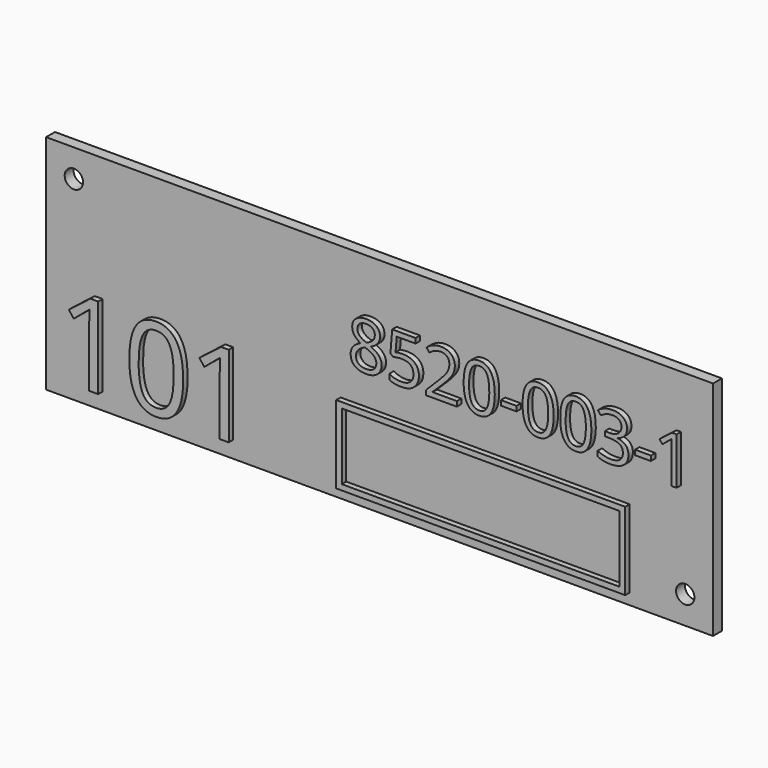
from build123d import *

# Parameters (mm, degrees)
F0_W         = 120
F0_H         = 40
F1_DEPTH     = 2
F3_D         = 3.3
F4_TEXT_SIZE = 11.8591723286
F5_DEPTH     = 1
F6_TEXT_SIZE = 20.5478077656
F7_DEPTH     = 1
F8_W         = 52
F8_H         = 14
F8_W_2       = 49.99999962
F8_H_2       = 11.99999962
F9_DEPTH     = 1


# Not quite as in the source:
# - Text() gives the source's letters only with a copy of the font that has no kerning and outlines rounded to 1/6400 em; it was checked with that copy


with BuildPart() as f1:
    # F0 (on Front) → F1 (new body)
    with BuildSketch(Plane.XZ):
        Rectangle(F0_W, F0_H)
    extrude(amount=F1_DEPTH)

    # F3 (through all)
    with Locations(Plane.XZ.offset(2)):
        with Locations((-55, 15), (55, -15)):
            Hole(F3_D / 2)

    # F4 (on face) → F5 (join)
    with BuildSketch(Plane.XZ.offset(2)):
        with Locations((-5, 2)):
            Text('8520-003-1', F4_TEXT_SIZE, font='Open Sans', text_align=(TextAlign.LEFT, TextAlign.BOTTOM))
    extrude(amount=F5_DEPTH)

    # F6 (on face) → F7 (join)
    with BuildSketch(Plane.XZ.offset(2)):
        with Locations((-57, -17)):
            Text('101', F6_TEXT_SIZE, font='Open Sans', text_align=(TextAlign.LEFT, TextAlign.BOTTOM))
    extrude(amount=F7_DEPTH)

    # F8 (on face) → F9 (join)
    with BuildSketch(Plane.XZ.offset(2)):
        with Locations((19, -11)):
            Rectangle(F8_W, F8_H)
        with Locations((19, -11)):
            Rectangle(F8_W_2, F8_H_2, mode=Mode.SUBTRACT)
    extrude(amount=F9_DEPTH)


solid = f1.part
